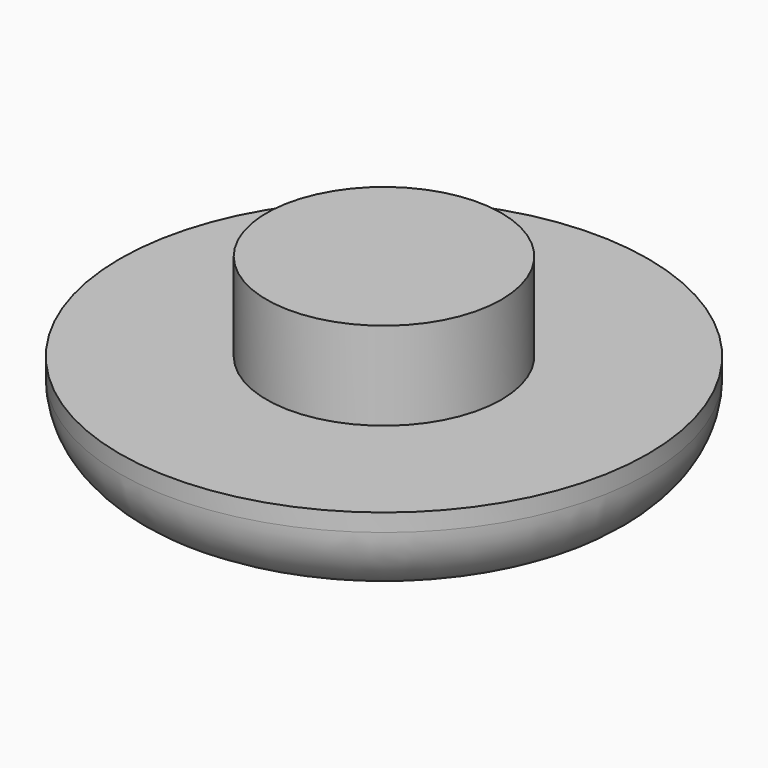
from build123d import *

# Parameters (mm, degrees)
F0_R         = 9
F1_DEPTH     = 3
F2_R         = 4
F3_DEPTH     = 3
F4_R         = 2.4
F5_TEXT_SIZE = 7.9588083219
F6_DEPTH     = 1.5


# Not quite as in the source:
# - Text() gives the source's letters only with a copy of the font that has no kerning and outlines rounded to 1/6400 em; it was checked with that copy


with BuildPart() as f1:
    # F0 (on Top) → F1 (new body)
    with BuildSketch(Plane.XY):
        Circle(F0_R)
    extrude(amount=F1_DEPTH)

    # F2 (on face) → F3 (join)
    with BuildSketch(Plane.XY.offset(3)):
        Circle(F2_R)
    extrude(amount=F3_DEPTH)

    # F4
    f4_edges = [f1.edges().sort_by_distance(p)[0] for p in [
        (-9, 0, 0),
    ]]
    fillet(f4_edges, radius=F4_R)

    # F5 (on face) → F6 (cut)
    with BuildSketch(Plane(origin=(0, 0, 0), x_dir=(1, 0, 0), z_dir=(0, 0, -1))):
        with Locations((-5.9751175252, -3.207139952)):
            Text('AM', F5_TEXT_SIZE, font='Open Sans', font_style=FontStyle.ITALIC, text_align=(TextAlign.LEFT, TextAlign.BOTTOM))
    extrude(amount=-F6_DEPTH, mode=Mode.SUBTRACT)


solid = f1.part
